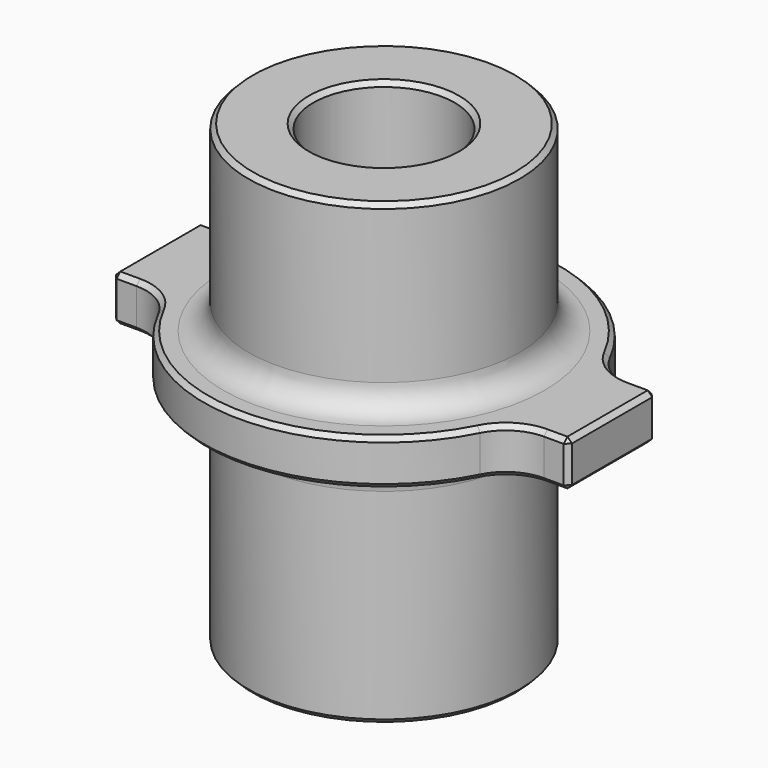
from build123d import *

# Parameters (mm, degrees)
F2_W     = 6.9
F2_H     = 4.8
F3_DEPTH = 2
F4_R     = 2.1
F5_SIZE  = 0.2
F6_R     = 1.1


# Not quite as in the source:
# - a feature names something its author has since deleted; it is built from what else it names


with BuildPart() as f1:
    # F0 (on Front) → F1 (revolve)
    with BuildSketch(Plane.XZ):
        Polygon((3.1, 0), (3.1, -12.1), (5.95, -12.1), (5.95, -2), (7.9, -2), (7.9, 0), (5.95, 0), (5.95, 8), (3.1, 8), align=None)
    revolve(axis=Axis((0, 0, -6.05), (0, 0, -1)))

    # F2 (on face) → F3 (join)
    with BuildSketch(Plane.XY):
        with Locations((6.55, 0)):
            Rectangle(F2_W, F2_H)
        with Locations((-6.55, 0)):
            Rectangle(F2_W, F2_H)
    extrude(amount=-F3_DEPTH)

    # F4
    f4_edges = [f1.edges().sort_by_distance(p)[0] for p in [
        (7.526619, -2.4, -1),
        (7.526619, 2.4, -1),
        (-7.526619, 2.4, -1),
        (-7.526619, -2.4, -1),
    ]]
    fillet(f4_edges, radius=F4_R)

    # F5
    f5_edges = [f1.edges().sort_by_distance(p)[0] for p in [
        (3.1, 0, -2.05),
        (-3.1, 0, -12.1),
        (-3.1, 0, 8),
        (-3.1, 0, -1),
        (10, -2.4, -1),
        (10, 2.4, -1),
        (10, 0, 0),
        (10, 0, -2),
        (0, -7.9, -2),
        (0, -7.9, 0),
        (9.465143, -2.4, 0),
        (9.465143, -2.4, -2),
        (9.465143, 2.4, 0),
        (9.465143, 2.4, -2),
        (-10, 2.4, -1),
        (-10, -2.4, -1),
        (-10, 0, 0),
        (-10, 0, -2),
        (-9.465143, -2.4, 0),
        (-9.465143, -2.4, -2),
        (-9.465143, 2.4, -2),
        (-9.465143, 2.4, 0),
        (-5.95, 0, 8),
        (-5.95, 0, -12.1),
        (7.829036, -2.711914, 0),
        (-7.829036, -2.711914, 0),
        (7.829036, 2.711914, 0),
        (0, 7.9, 0),
        (-7.829036, 2.711914, 0),
        (7.829036, -2.711914, -2),
        (-7.829036, -2.711914, -2),
        (7.829036, 2.711914, -2),
        (0, 7.9, -2),
        (-7.829036, 2.711914, -2),
    ]]
    chamfer(f5_edges, length=F5_SIZE)

    # F6
    f6_edges = [f1.edges().sort_by_distance(p)[0] for p in [
        (-5.95, 0, -2),
        (-5.95, 0, 0),
    ]]
    fillet(f6_edges, radius=F6_R)


solid = f1.part
